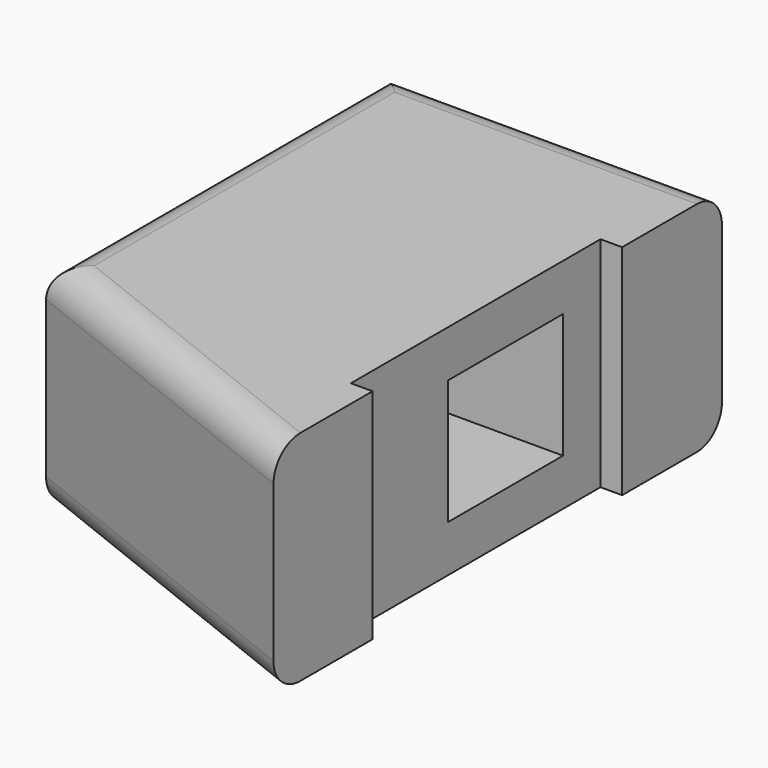
from build123d import *

# Parameters (mm, degrees)
F0_W         = 170
F0_H         = 18
F0_TEXT_SIZE = 13.8888888889
F1_DEPTH     = 3.5
F3_DEPTH     = 2
F5_DEPTH     = 7.5
F6_R         = 1
F7_W         = 160.9919443727
F7_H         = 25.8382139727
F8_DEPTH     = 12.5


# Not quite as in the source:
# - Text() gives the source's letters only with a copy of the font that has no kerning and outlines rounded to 1/6400 em; it was checked with that copy


with BuildPart() as f1:
    # F0 (on Top) → F1 (new body, symmetric)
    with BuildSketch(Plane.XY):
        with Locations((-30.7142301194, 0)):
            Rectangle(F0_W, F0_H)
        Polygon((-105.7142301194, -5), (-105.7142301194, 5), (50.2857698806, 5), (50.2857698806, -5), (44.3851622417, -5), (41.9849886306, -5), (37.3734434917, -5), (35.120839325, -5), (32.855214325, -5), (27.8031309917, -5), (25.5375059917, -5), (24.2896761306, -5), (22.3300407139, -5), (19.8148497417, -5), (17.8877664084, -5), (15.570058075, -5), (13.6907177972, -5), (8.8339469639, -5), (6.4337733528, -5), (1.8222282139, -5), (-0.4303759528, -5), (-2.6960009528, -5), (-7.7480842861, -5), (-10.0137092861, -5), (-11.2615391472, -5), (-13.2211745639, -5), (-15.7363655361, -5), (-17.6634488694, -5), (-19.9811572028, -5), (-21.8604974805, -5), (-26.7172683139, -5), (-29.117441925, -5), (-33.7289870639, -5), (-35.9815912305, -5), (-38.2472162305, -5), (-43.2992995639, -5), (-45.5649245639, -5), (-46.812754425, -5), (-48.7723898416, -5), (-51.2875808139, -5), (-53.2146641472, -5), (-55.5323724805, -5), (-57.4117127583, -5), (-62.2684835916, -5), (-64.6686572028, -5), (-69.2802023416, -5), (-71.5328065083, -5), (-73.7984315083, -5), (-78.8505148416, -5), (-81.1161398416, -5), (-82.3639697028, -5), (-84.3236051194, -5), (-86.8387960916, -5), (-88.765879425, -5), (-91.0835877583, -5), (-92.9629280361, -5), align=None, mode=Mode.SUBTRACT)
        with Locations((-94.2107578972, -5)):
            Text('MAX MAX MAX MAX', F0_TEXT_SIZE, font='Open Sans', font_style=FontStyle.BOLD, text_align=(TextAlign.LEFT, TextAlign.BOTTOM))
    extrude(amount=F1_DEPTH, both=True)

    # F2 (on Top) → F3 (cut, symmetric)
    with BuildSketch(Plane.XY):
        Polygon((-105.2142301194, 3.5), (-116.7142301194, 3.5), (-116.7142301194, -3.5), (-105.2142301194, -1), align=None)
    extrude(amount=F3_DEPTH, both=True, mode=Mode.SUBTRACT)

    # F4 (on Top) → F5 (cut, symmetric)
    with BuildSketch(Plane.XY):
        Polygon((-117.7709698677, -10.5618461967), (-104.4237911701, -9.2072207481), (-117.7709698677, -3.8991386537), align=None)
    extrude(amount=F5_DEPTH, both=True, mode=Mode.SUBTRACT)

    # F6
    f6_edges = [f1.edges().sort_by_distance(p)[0] for p in [
        (54.28577, 0, -3.5),
        (-30.71423, 9, -3.5),
        (-25.329539, -9, -3.5),
        (54.28577, 0, 3.5),
        (54.28577, 9, 0),
        (54.28577, -9, 0),
        (-110.329539, -6.858545, -3.5),
        (-25.329539, -9, 3.5),
        (-30.71423, 9, 3.5),
        (-115.71423, 2.141455, 3.5),
        (-110.329539, -6.858545, 3.5),
    ]]
    fillet(f6_edges, radius=F6_R)

    # F7 (on Top) → F8 (cut, symmetric)
    with BuildSketch(Plane.XY):
        with Locations((-24.5246551931, -0.8951523341)):
            Rectangle(F7_W, F7_H)
    extrude(amount=F8_DEPTH, both=True, mode=Mode.SUBTRACT)


solid = f1.part
